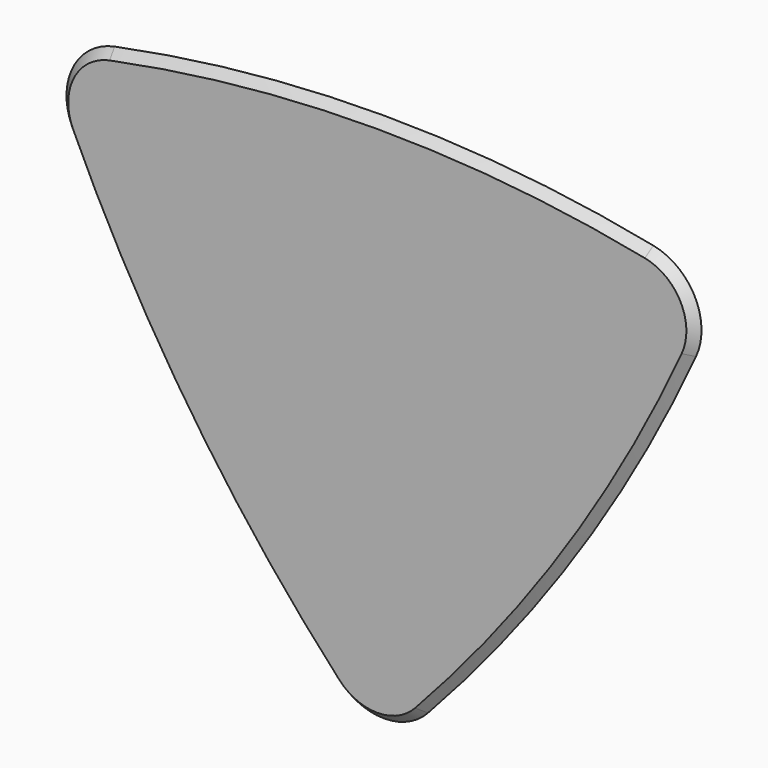
from build123d import *

# Parameters (mm, degrees)
F1_DEPTH = 1.778
F2_SIZE  = 1.77799


# Not quite as in the source:
# - a fillet or chamfer is up to 0.001 mm smaller than in the source, because OpenCascade refuses the exact size


with BuildPart() as f1:
    # F0 (on Front) → F1 (new body)
    with BuildSketch(Plane.XZ):
        with BuildLine():
            ThreePointArc((66.0201128793, 29.4303813325), (65.7972189254, 40.488980065), (56.9887202123, 47.1787213202))
            ThreePointArc((56.9887202123, 47.1787213202), (-0.0054733282, 52.8677532198), (-56.9996870512, 47.1789235179))
            ThreePointArc((-56.9996870512, 47.1789235179), (-65.8085669907, 40.4885109251), (-66.0304847763, 29.4291827833))
            ThreePointArc((-66.0304847763, 29.4291827833), (-41.0456047225, -15.2401883532), (-9.3070649286, -55.3931713157))
            ThreePointArc((-9.3070649286, -55.3931713157), (0.0001097607, -59.4518124354), (9.3070583612, -55.392652894))
            ThreePointArc((9.3070583612, -55.392652894), (41.0411349867, -15.2393801728), (66.0201128793, 29.4303813325))
        make_face()
    extrude(amount=F1_DEPTH)

    # F2 (size 1.778 in the source; OpenCascade refuses exactly that, so slightly less here)
    f2_edges = [f1.edges().sort_by_distance(p)[0] for p in [
        (-41.045605, -1.778, -15.240188),
    ]]
    chamfer(f2_edges, length=F2_SIZE)


solid = f1.part
